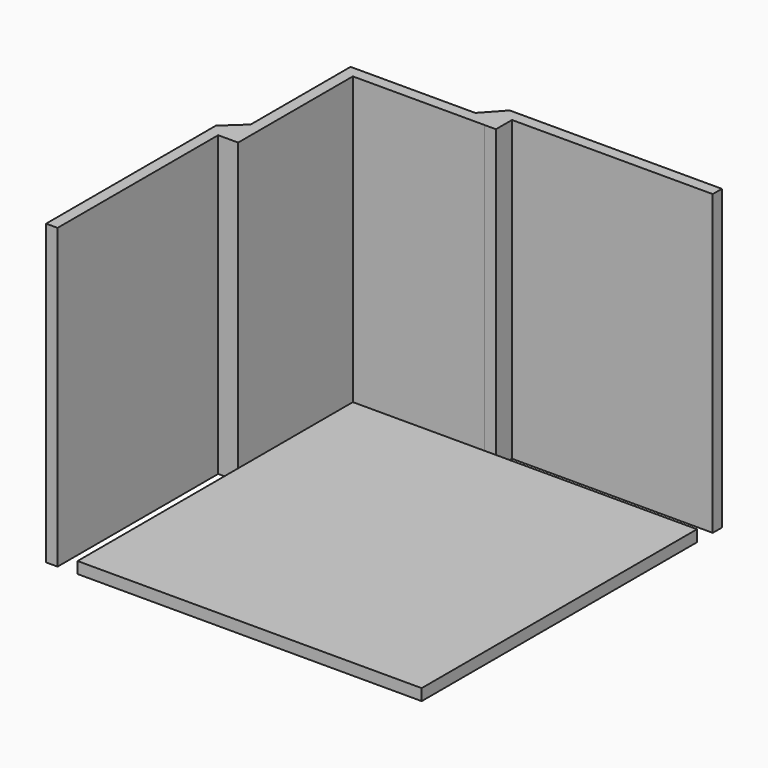
from build123d import *

# Parameters (mm, degrees)
F0_W     = 30
F0_H     = 30
F1_DEPTH = 2
F0_W_2   = 2
F0_H_2   = 1.9999989867
F0_W_3   = 1.9999989867
F0_H_3   = 2
F2_DEPTH = 52


with BuildPart() as f1:
    # F0 (on Top) → F1 (new body)
    with BuildSketch(Plane.XY):
        Polygon((-11.9309425354, 30.1818712056), (-29.8587139696, 30.1818712056), (-29.8587139696, 12.2573869303), (-29.8587139696, 7.1818712056), (-29.8587139696, 5.1818712056), (-29.8587139696, 0.1818712056), (0.1412860304, 0.1818712056), (0.1412860304, 30.1818712056), (-4.8587139696, 30.1818712056), (-4.9099967368, 30.1818712056), (-6.9099967368, 30.1818712056), align=None)
        Polygon((0.1412860304, 0.1818712056), (-29.8587139696, 0.1818712056), (-29.8587139696, -29.8181287944), (-29.847416997, -29.8181287944), (0.1412860304, -29.8181287944), align=None)
        Polygon((30.0900032632, 30.1818712056), (0.1412860304, 30.1818712056), (0.1412860304, 0.1818712056), (30.1412860304, 0.1818712056), (30.1412860304, 30.1818712056), align=None)
        with Locations((15.1412860304, -14.8181287944)):
            Rectangle(F0_W, F0_H)
    extrude(amount=F1_DEPTH)

    # F0 (on Top) → F2 (join)
    with BuildSketch(Plane.XY):
        Polygon((-31.8587129563, 5.1818712056), (-31.8587129563, 7.1818712056), (-35.347416997, 7.1818712056), (-35.347416997, -29.8181287944), (-33.347416997, -29.8181287944), (-33.347416997, 5.1818712056), align=None)
        with Locations((-5.9099967368, 31.1818706989)):
            Rectangle(F0_W_2, F0_H_2)
        Polygon((-6.9099967368, 35.6818712056), (-10.1051449882, 32.1818701923), (-6.9099967368, 32.1818701923), align=None)
        Polygon((-31.8587129563, 7.1818712056), (-31.8587129563, 10.4079470433), (-35.347416997, 7.1818712056), align=None)
        Polygon((-10.1051449882, 32.1818701923), (-11.9309425354, 30.1818712056), (-6.9099967368, 30.1818712056), (-6.9099967368, 32.1818701923), align=None)
        Polygon((-6.9099967368, 35.6818712056), (-6.9099967368, 32.1818701923), (-4.9099967368, 32.1818701923), (-4.9099967368, 33.6818712056), (30.0900032632, 33.6818712056), (30.0900032632, 35.6818712056), align=None)
        Polygon((-29.8587139696, 12.2573869303), (-29.8587139696, 30.1818712056), (-11.9309425354, 30.1818712056), (-10.1051449882, 32.1818701923), (-31.8587129563, 32.1818701923), (-31.8587129563, 10.4079470433), align=None)
        Polygon((-29.8587139696, 7.1818712056), (-29.8587139696, 12.2573869303), (-31.8587129563, 10.4079470433), (-31.8587129563, 7.1818712056), align=None)
        with Locations((-30.8587134629, 6.1818712056)):
            Rectangle(F0_W_3, F0_H_3)
    extrude(amount=F2_DEPTH)


solid = f1.part
